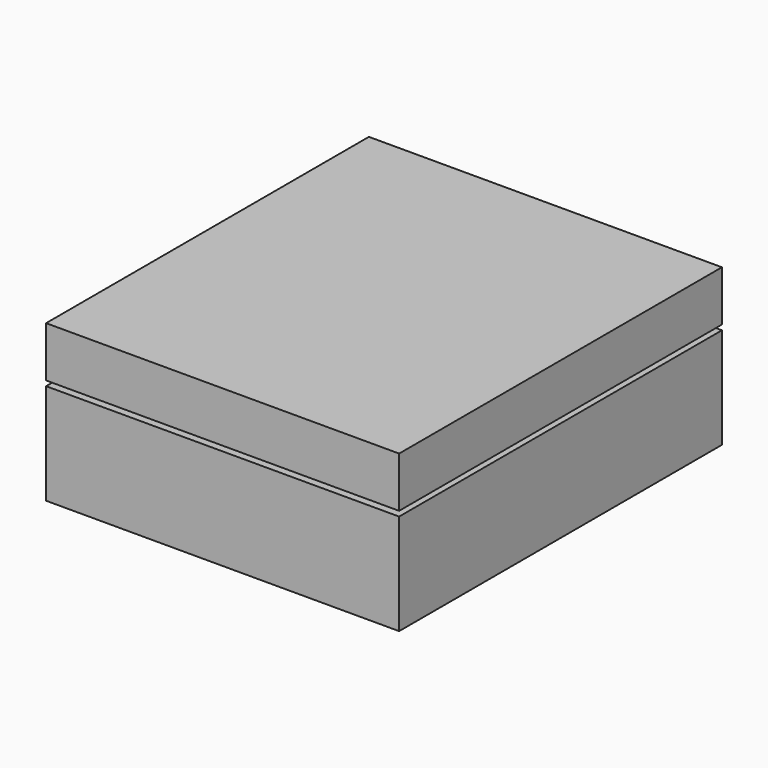
from build123d import *

# Parameters (mm, degrees)
F0_W     = 35
F0_H     = 40
F1_DEPTH = 10
F3_DEPTH = 5
F5_W     = 35
F5_H     = 40
F6_DEPTH = 5


with BuildPart() as f1:
    # F0 (on Top) → F1 (new body)
    with BuildSketch(Plane.XY):
        Rectangle(F0_W, F0_H)
    extrude(amount=F1_DEPTH)

    # F2 (on face) → F3 (cut)
    with BuildSketch(Plane.XY.offset(10)):
        Polygon((-12.5, -15), (12.5, -15), (12.5, 11.5108080208), (9.5269214362, 15), (-12.5, 15), align=None)
    extrude(amount=-F3_DEPTH, mode=Mode.SUBTRACT)


with BuildPart() as f6:
    # F5 (on offset) → F6 (new body)
    with BuildSketch(Plane.XY.offset(10.5)):
        Rectangle(F5_W, F5_H)
    extrude(amount=F6_DEPTH)


solid = Compound([f1.part, f6.part])
